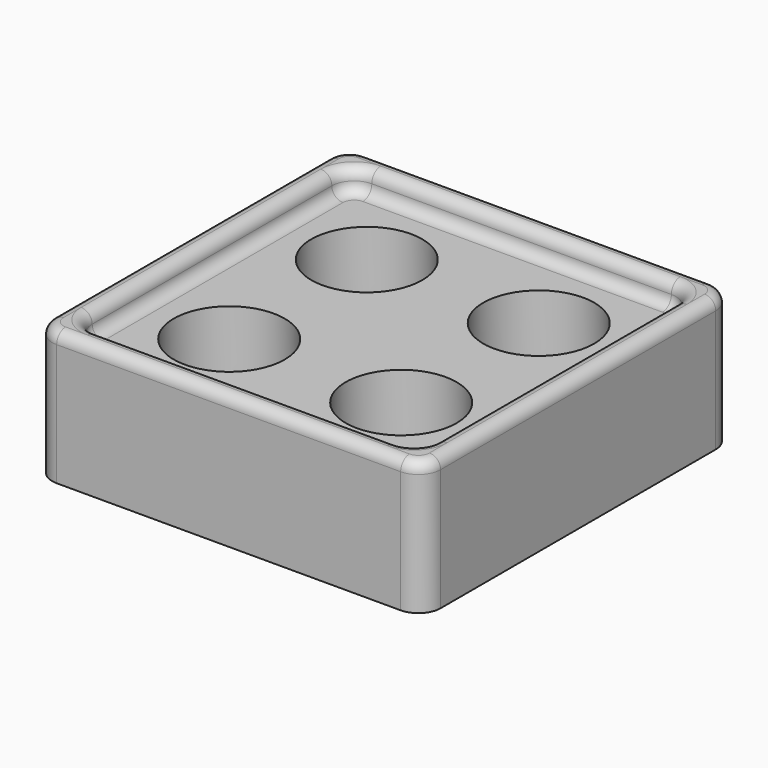
from build123d import *

# Parameters (mm, degrees)
F0_W     = 19.685
F0_H     = 19.685
F0_R     = 3.175
F1_DEPTH = 7.62
F2_DEPTH = 1.27
F3_DEPTH = 6.0452
F4_R     = 1.27
F5_R     = 0.63499


# Not quite as in the source:
# - a fillet or chamfer is up to 0.001 mm smaller than in the source, because OpenCascade refuses the exact size


with BuildPart() as f1:
    # F0 (on Top) → F1 (new body)
    with BuildSketch(Plane.XY):
        Polygon((-11.1125, 11.1125), (-9.8425, 9.8425), (9.8425, 9.8425), (11.1125, 11.1125), align=None)
        Polygon((11.1125, 11.1125), (9.8425, 9.8425), (9.8425, -9.8425), (11.1125, -11.1125), align=None)
        Polygon((-9.8425, -9.8425), (-9.8425, 9.8425), (-11.1125, 11.1125), (-11.1125, -11.1125), align=None)
        Polygon((9.8425, -9.8425), (-9.8425, -9.8425), (-11.1125, -11.1125), (11.1125, -11.1125), align=None)
        Rectangle(F0_W, F0_H)
        with Locations((-4.92125, -4.92125)):
            Circle(F0_R, mode=Mode.SUBTRACT)
        with Locations((4.92125, -4.92125)):
            Circle(F0_R, mode=Mode.SUBTRACT)
        with Locations((-4.92125, 4.92125)):
            Circle(F0_R, mode=Mode.SUBTRACT)
        with Locations((4.92125, 4.92125)):
            Circle(F0_R, mode=Mode.SUBTRACT)
        with Locations((-4.92125, 4.92125)):
            Circle(F0_R)
        with Locations((4.92125, 4.92125)):
            Circle(F0_R)
        with Locations((-4.92125, -4.92125)):
            Circle(F0_R)
        with Locations((4.92125, -4.92125)):
            Circle(F0_R)
    extrude(amount=-F1_DEPTH)

    # F0 (on Top) → F2 (cut)
    with BuildSketch(Plane.XY):
        Rectangle(F0_W, F0_H)
        with Locations((-4.92125, -4.92125)):
            Circle(F0_R, mode=Mode.SUBTRACT)
        with Locations((4.92125, -4.92125)):
            Circle(F0_R, mode=Mode.SUBTRACT)
        with Locations((-4.92125, 4.92125)):
            Circle(F0_R, mode=Mode.SUBTRACT)
        with Locations((4.92125, 4.92125)):
            Circle(F0_R, mode=Mode.SUBTRACT)
        with Locations((-4.92125, 4.92125)):
            Circle(F0_R)
        with Locations((4.92125, 4.92125)):
            Circle(F0_R)
        with Locations((4.92125, -4.92125)):
            Circle(F0_R)
        with Locations((-4.92125, -4.92125)):
            Circle(F0_R)
    extrude(amount=-F2_DEPTH, mode=Mode.SUBTRACT)

    # F0 (on Top) → F3 (cut)
    with BuildSketch(Plane.XY):
        with Locations((-4.92125, 4.92125)):
            Circle(F0_R)
        with Locations((-4.92125, -4.92125)):
            Circle(F0_R)
        with Locations((4.92125, -4.92125)):
            Circle(F0_R)
        with Locations((4.92125, 4.92125)):
            Circle(F0_R)
    extrude(amount=-F3_DEPTH, mode=Mode.SUBTRACT)

    # F4
    f4_edges = [f1.edges().sort_by_distance(p)[0] for p in [
        (11.1125, -11.1125, -3.81),
        (11.1125, 11.1125, -3.81),
        (-11.1125, -11.1125, -3.81),
        (-11.1125, 11.1125, -3.81),
        (-9.8425, -9.8425, -0.635),
        (-9.8425, 9.8425, -0.635),
        (9.8425, 9.8425, -0.635),
        (9.8425, -9.8425, -0.635),
    ]]
    fillet(f4_edges, radius=F4_R)

    # F5 (radius 0.635 in the source; OpenCascade refuses exactly that, so slightly less here)
    f5_edges = [f1.edges().sort_by_distance(p)[0] for p in [
        (-8.09625, 4.92125, -6.0452),
        (1.74625, 4.92125, -6.0452),
        (1.74625, -4.92125, -6.0452),
        (-8.09625, -4.92125, -6.0452),
        (-9.8425, 0, -1.27),
        (0, 9.8425, 0),
        (-11.1125, 0, 0),
    ]]
    fillet(f5_edges, radius=F5_R)


solid = f1.part
